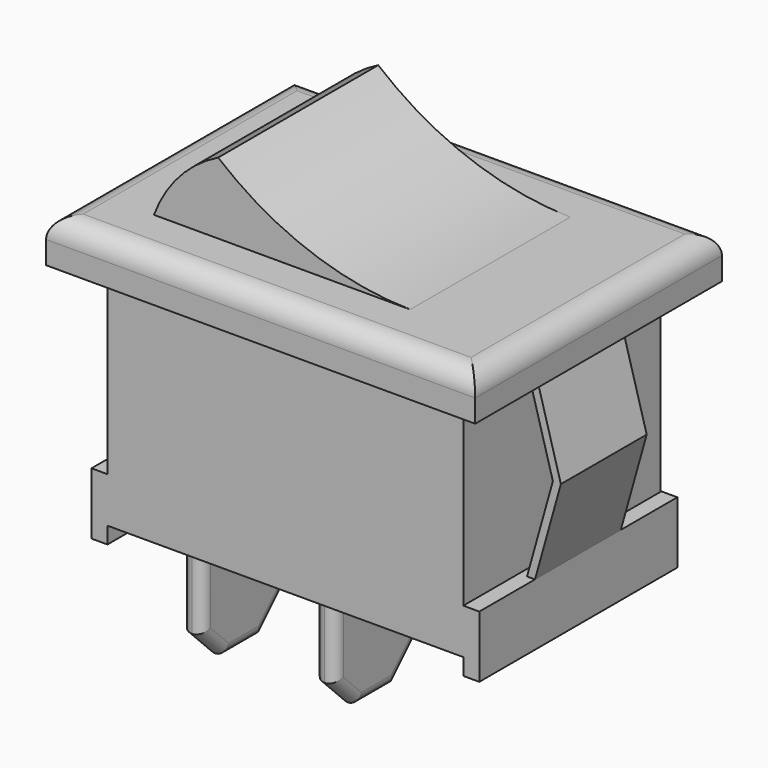
from build123d import *

# Parameters (mm, degrees)
F0_W      = 17.25
F0_H      = 10.95
F1_DEPTH  = 5.975
F3_DEPTH  = 12
F4_W      = 17.25
F4_H      = 0.8041968666
F5_DEPTH  = 12.001
F7_DEPTH  = 2.6
F9_DEPTH  = 7.475
F10_W     = 1
F10_H     = 5
F11_DEPTH = 7
F12_SIZE  = 1.4
F13_R     = 0.49999
F14_R     = 1
F16_DEPTH = 4.85


# Not quite as in the source:
# - a fillet or chamfer is up to 0.001 mm smaller than in the source, because OpenCascade refuses the exact size


with BuildPart() as f1:
    # F0 (on Front) → F1 (new body, symmetric)
    with BuildSketch(Plane.XZ):
        Rectangle(F0_W, F0_H)
    extrude(amount=F1_DEPTH, both=True)

    # F2 (on face) → F3 (join)
    with BuildSketch(Plane.XZ.offset(5.975)):
        Polygon((-8.625, -5.475), (8.625, -5.475), (8.625, -3.475), (0, -3.475), (-8.625, -3.475), align=None)
        Polygon((8.625, -3.475), (8.625, -5.475), (-8.625, -5.475), (-8.625, -3.475), (-9.4, -3.475), (-9.4, -6.475), (0, -6.475), (9.4, -6.475), (9.4, -3.475), align=None)
    extrude(amount=-F3_DEPTH)

    # F4 (on face) → F5 (cut, through all)
    with BuildSketch(Plane.XZ.offset(5.975)):
        with Locations((0, -6.0729015667)):
            Rectangle(F4_W, F4_H)
    extrude(amount=-F5_DEPTH, mode=Mode.SUBTRACT)

    # F6 (on Front) → F7 (join, symmetric)
    with BuildSketch(Plane.XZ):
        Polygon((-10.653115809, 1), (-9.4, -3.475), (-9.0125, -3.475), (-10.265615809, 1), (-9.0125, 5.475), (-9.4, 5.475), align=None)
        Polygon((10.265615809, 1), (9.0125, -3.475), (9.4, -3.475), (10.653115809, 1), (9.4, 5.475), (9.0125, 5.475), align=None)
    extrude(amount=F7_DEPTH, both=True)

    # F8 (on Front) → F9 (join, symmetric)
    with BuildSketch(Plane.XZ):
        Polygon((-10.4, 5.475), (-8.625, 5.475), (8.625, 5.475), (10.4, 5.475), (10.4, 7.575), (-10.4, 7.575), align=None)
    extrude(amount=F9_DEPTH, both=True)

    # F10 (on face) → F11 (join)
    with BuildSketch(Plane(origin=(0, 0, -5.6708031334), x_dir=(1, 0, 0), z_dir=(0, 0, -1))):
        with Locations((-7.3124970421, 0)):
            Rectangle(F10_W, F10_H)
        with Locations((-0.875, 0)):
            Rectangle(F10_W, F10_H)
    extrude(amount=F11_DEPTH)

    # F12
    f12_edges = [f1.edges().sort_by_distance(p)[0] for p in [
        (-7.312497, -2.5, -12.670803),
        (-7.312497, 2.5, -12.670803),
        (-0.875, -2.5, -12.670803),
        (-0.875, 2.5, -12.670803),
    ]]
    chamfer(f12_edges, length=F12_SIZE)

    # F13 (radius 0.5 in the source; OpenCascade refuses exactly that, so slightly less here)
    f13_edges = [f1.edges().sort_by_distance(p)[0] for p in [
        (-6.812497, -2.5, -8.470803),
        (-7.812497, -2.5, -8.470803),
        (-6.812497, -1.8, -11.970803),
        (-7.812497, -1.8, -11.970803),
        (-6.812497, 0, -12.670803),
        (-7.812497, 0, -12.670803),
        (-6.812497, 1.8, -11.970803),
        (-7.812497, 1.8, -11.970803),
        (-6.812497, 2.5, -8.470803),
        (-7.812497, 2.5, -8.470803),
        (-0.375, 2.5, -8.470803),
        (-1.375, 2.5, -8.470803),
        (-0.375, 1.8, -11.970803),
        (-1.375, 1.8, -11.970803),
        (-0.375, 0, -12.670803),
        (-1.375, 0, -12.670803),
        (-0.375, -1.8, -11.970803),
        (-1.375, -1.8, -11.970803),
        (-0.375, -2.5, -8.470803),
        (-1.375, -2.5, -8.470803),
    ]]
    fillet(f13_edges, radius=F13_R)

    # F14
    f14_edges = [f1.edges().sort_by_distance(p)[0] for p in [
        (0, -7.475, 7.575),
        (10.4, 0, 7.575),
        (0, 7.475, 7.575),
        (-10.4, 0, 7.575),
    ]]
    fillet(f14_edges, radius=F14_R)

    # F15 (on Front) → F16 (join, symmetric)
    with BuildSketch(Plane.XZ):
        with BuildLine():
            ThreePointArc((-4.1594156064, 11.0315568745), (-6.0465979045, 9.6017056311), (-7.2706877254, 7.575))
            Line((-7.2706877254, 7.575), (5.1499965846, 7.575))
            ThreePointArc((5.1499965846, 7.575), (0.2006102654, 8.5096274816), (-4.1594156064, 11.0315568745))
        make_face()
    extrude(amount=F16_DEPTH, both=True)


solid = f1.part
